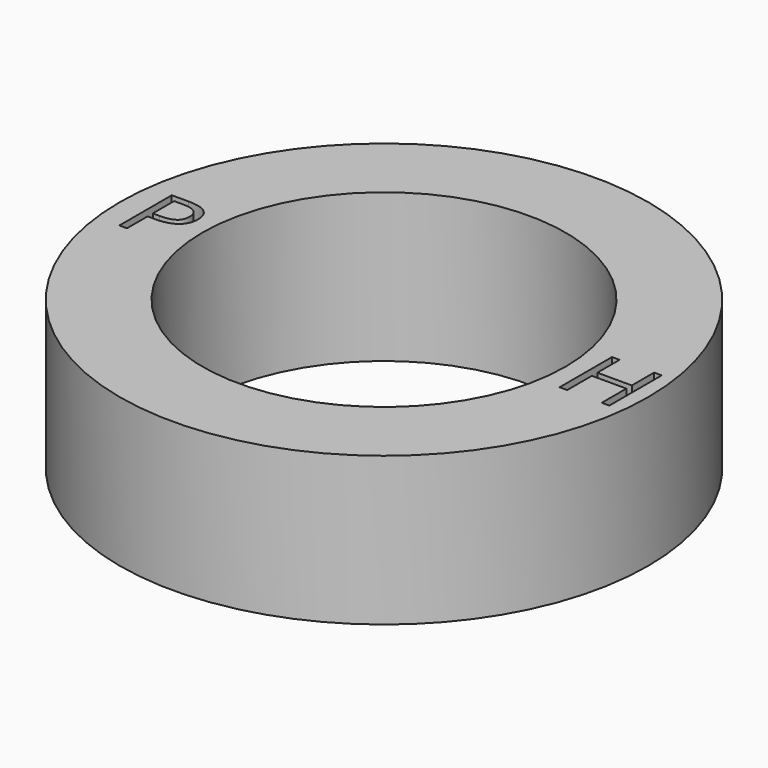
from build123d import *

# Parameters (mm, degrees)
F0_R         = 16
F2_DEPTH     = 9
F1_R         = 11
F3_DEPTH     = 74.168
F4_TEXT_SIZE = 5.5555555556
F5_DEPTH     = 50
F6_TEXT_SIZE = 5.5555555556
F7_DEPTH     = 25


# Not quite as in the source:
# - Text() gives the source's letters only with a copy of the font that has no kerning and outlines rounded to 1/6400 em; it was checked with that copy


with BuildPart() as f2:
    # F0 (on Top) → F2 (new body)
    with BuildSketch(Plane.XY):
        Circle(F0_R)
    extrude(amount=F2_DEPTH)

    # F1 (on Top) → F3 (cut)
    with BuildSketch(Plane.XY):
        Circle(F1_R)
    extrude(amount=F3_DEPTH, mode=Mode.SUBTRACT)

    # F4 (on Top) → F5 (cut)
    with BuildSketch(Plane.XY):
        with Locations((-15.0655200825, -1.8883662215)):
            Text('P', F4_TEXT_SIZE, font='Open Sans', text_align=(TextAlign.LEFT, TextAlign.BOTTOM))
    extrude(amount=F5_DEPTH, mode=Mode.SUBTRACT)

    # F6 (on Top) → F7 (cut)
    with BuildSketch(Plane.XY):
        with Locations((11.5494824159, -1.8196424801)):
            Text('H', F6_TEXT_SIZE, font='Open Sans', text_align=(TextAlign.LEFT, TextAlign.BOTTOM))
    extrude(amount=F7_DEPTH, mode=Mode.SUBTRACT)


solid = f2.part
